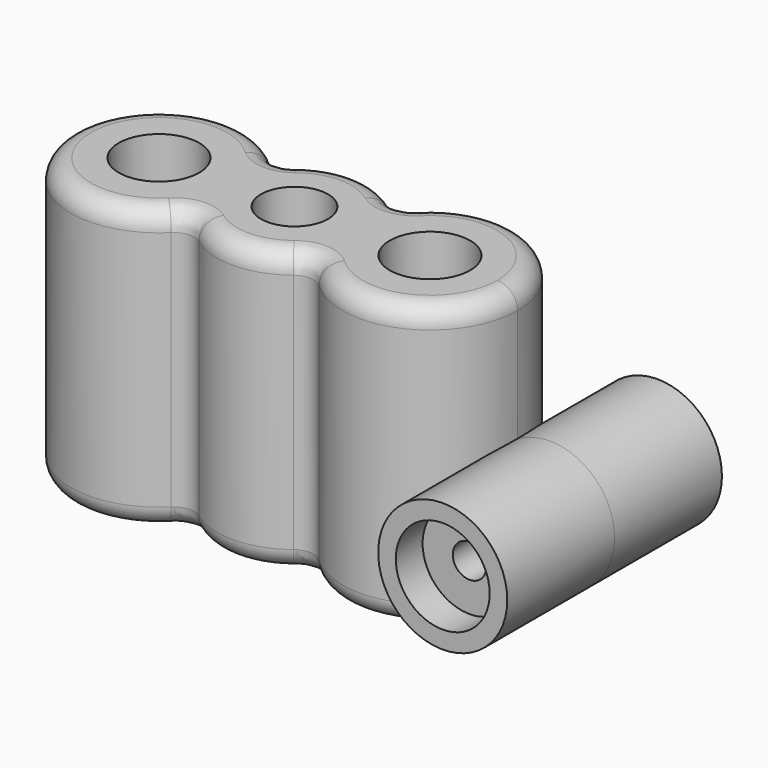
from build123d import *

# Parameters (mm, degrees)
F1_DEPTH       = 42
F2_R           = 9.6174487521
F3_DEPTH       = 20
F4_DEPTH       = 20
F5_D           = 12
F6_D           = 10
F8_D           = 5
F8_CBORE_D     = 14
F8_CBORE_DEPTH = 5
F9_F1_R        = 3
F9_F2_R        = 3


# Not quite as in the source:
# - a feature names something its author has since deleted; it is built from what else it names


with BuildPart() as f1:
    # F0 (on Top) → F1 (new body)
    with BuildSketch(Plane.XY):
        with BuildLine():
            ThreePointArc((9.1505627454, -7.0033062659), (23.7868709109, -12.2415465763), (33.0476022533, 0.2444268846))
            ThreePointArc((33.0476022533, 0.2444268846), (23.6340041516, 12.7757451866), (8.9766756052, 7.2248454857))
            ThreePointArc((8.9766756052, 7.2248454857), (10.8677771882, 3.8302109864), (11.5229812641, 0))
            ThreePointArc((11.5229812641, 0), (10.9137724982, -3.6971160477), (9.1505627454, -7.0033062659))
        make_face()
        with BuildLine():
            ThreePointArc((11.5229812641, 0), (10.8677771882, 3.8302109864), (8.9766756052, 7.2248454857))
            ThreePointArc((8.9766756052, 7.2248454857), (6.9533720407, 0.0849795533), (9.1505627454, -7.0033062659))
            ThreePointArc((9.1505627454, -7.0033062659), (10.9137724982, -3.6971160477), (11.5229812641, 0))
        make_face()
        with BuildLine():
            ThreePointArc((9.1505627454, -7.0033062659), (6.9533720407, 0.0849795533), (8.9766756052, 7.2248454857))
            ThreePointArc((8.9766756052, 7.2248454857), (-0.0835171314, 11.5226785992), (-9.0804592928, 7.0939661858))
            ThreePointArc((-9.0804592928, 7.0939661858), (-7.415302968, 3.5914280039), (-6.8436942073, -0.2444268846))
            ThreePointArc((-6.8436942073, -0.2444268846), (-7.3693668934, -3.9262049114), (-8.9043774496, -7.3137650665))
            ThreePointArc((-8.9043774496, -7.3137650665), (0.1981109959, -11.5212781082), (9.1505627454, -7.0033062659))
        make_face()
        with BuildLine():
            ThreePointArc((-6.8436942073, -0.2444268846), (-7.415302968, 3.5914280039), (-9.0804592928, 7.0939661858))
            ThreePointArc((-9.0804592928, 7.0939661858), (-11.522120817, -0.1408158047), (-8.9043774496, -7.3137650665))
            ThreePointArc((-8.9043774496, -7.3137650665), (-7.3693668934, -3.9262049114), (-6.8436942073, -0.2444268846))
        make_face()
        with BuildLine():
            ThreePointArc((-8.9043774496, -7.3137650665), (-11.522120817, -0.1408158047), (-9.0804592928, 7.0939661858))
            ThreePointArc((-9.0804592928, 7.0939661858), (-33.1553233816, -0.40520262), (-8.9043774496, -7.3137650665))
        make_face()
    extrude(amount=F1_DEPTH)

    # F2 (on Front) → F3 (join)
    with BuildSketch(Plane.XZ):
        with Locations((38.0958206952, 14.0142505988)):
            Circle(F2_R)
    extrude(amount=F3_DEPTH)

    # F2 (on Front) → F4 (join)
    with BuildSketch(Plane.XZ):
        with Locations((38.0958206952, 14.0142505988)):
            Circle(F2_R)
    extrude(amount=-F4_DEPTH)

    # F5 (through all)
    with Locations(Plane(origin=(0, 0, 0), x_dir=(1, 0, 0), z_dir=(0, 0, -1))):
        with Locations((-20, 0.2444268846), (20, -0.2444268846)):
            Hole(F5_D / 2)

    # F6 (through all)
    with Locations(Plane(origin=(0, 0, 0), x_dir=(1, 0, 0), z_dir=(0, 0, -1))):
        with Locations((0, 0)):
            Hole(F6_D / 2)

    # F8 (through all)
    with Locations(Plane.XZ.offset(20)):
        with Locations((38.0958206952, 14.0142505988)):
            CounterBoreHole(F8_D / 2, F8_CBORE_D / 2, F8_CBORE_DEPTH)

    # F9: fillet of radius 3 on 8 edges, made by hand

    # F9_f1
    f9_f1_edges = [f1.edges().sort_by_distance(p)[0] for p in [
        (-8.9043774496, -7.3137650665, 21),
        (9.1505627454, -7.0033062659, 21),
        (8.9766756052, 7.2248454857, 21),
        (-9.0804592928, 7.0939661858, 21),
    ]]
    fillet(f9_f1_edges, radius=F9_F1_R)

    # F9_f2
    f9_f2_edges = [f1.edges().sort_by_distance(p)[0] for p in [
        (0.1844290224, -11.5215052466, 0),
        (0.1844290224, -11.5215052466, 42),
        (-0.0972005694, 11.5225712956, 0),
        (-0.0972005694, 11.5225712956, 42),
        (8.9038484363, 8.6404608623, 42),
        (-9.0385400019, 8.4885169801, 42),
        (8.9038484363, 8.6404608623, 0),
        (-9.0385400019, 8.4885169801, 0),
        (-8.8283891992, -8.7068748722, 42),
        (9.112353607, -8.4202786555, 42),
        (-8.8283891992, -8.7068748722, 0),
        (9.112353607, -8.4202786555, 0),
    ]]
    fillet(f9_f2_edges, radius=F9_F2_R)


solid = f1.part
